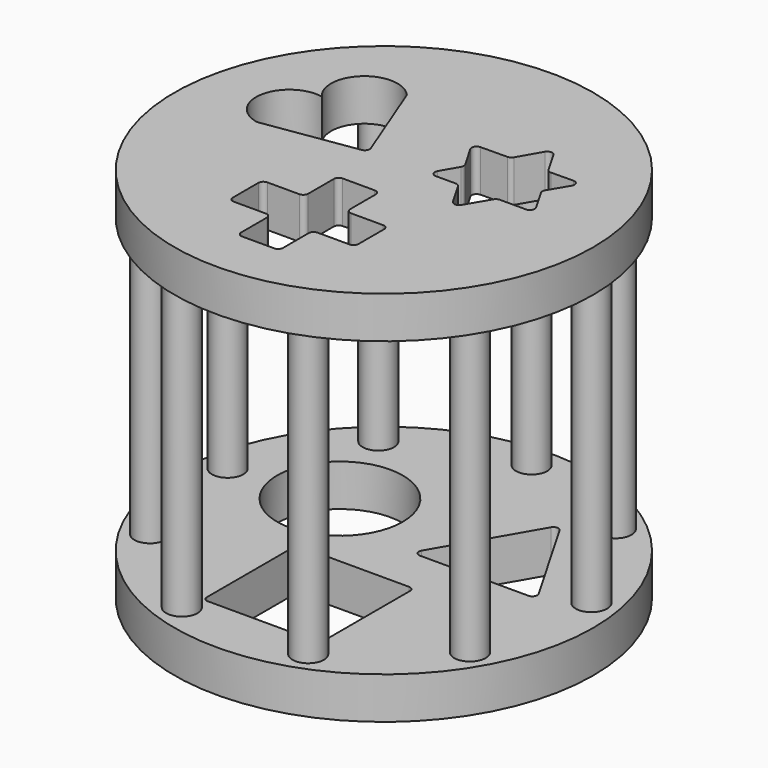
from build123d import *

# Parameters (mm, degrees)
F0_R      = 63.5
F0_R_2    = 19.05
F1_DEPTH  = 12.7
F2_R      = 4.7625
F3_DEPTH  = 6.35
F4_R      = 4.7625
F5_DEPTH  = 101.6
F7_COUNT  = 9
F7_ANGLE  = 320
F9_R      = 63.5
F10_DEPTH = 12.7
F11_R     = 4.7625
F12_DEPTH = 6.35


# Not quite as in the source:
# - a length typed as a fraction of an inch, garbled in the dataset ("3 / 203.2 mm" for 3/8 in), is restored


with BuildPart() as f1:
    # F0 (on Top) → F1 (new body)
    with BuildSketch(Plane.XY):
        Circle(F0_R)
        with BuildLine():
            Line((-17.78, -44.855), (-17.78, -12.295))
            ThreePointArc((-17.78, -12.295), (-17.3406601718, -11.2343398282), (-16.28, -10.795))
            Line((-16.28, -10.795), (16.28, -10.795))
            ThreePointArc((16.28, -10.795), (17.3406601718, -11.2343398282), (17.78, -12.295))
            Line((17.78, -12.295), (17.78, -44.855))
            ThreePointArc((17.78, -44.855), (17.3406601718, -45.9156601718), (16.28, -46.355))
            Line((16.28, -46.355), (-16.28, -46.355))
            ThreePointArc((-16.28, -46.355), (-17.3406601718, -45.9156601718), (-17.78, -44.855))
        make_face(mode=Mode.SUBTRACT)
        with Locations((-24.7466759131, 14.2875)):
            Circle(F0_R_2, mode=Mode.SUBTRACT)
        with BuildLine():
            ThreePointArc((8.2947521245, 3.2889773719), (6.9957140188, 4.0389773719), (6.9957140188, 5.5389773719))
            Line((6.9957140188, 5.5389773719), (23.4476378075, 34.0345452561))
            ThreePointArc((23.4476378075, 34.0345452561), (24.7466759131, 34.7845452561), (26.0457140188, 34.0345452561))
            Line((26.0457140188, 34.0345452561), (42.4976378075, 5.5389773719))
            ThreePointArc((42.4976378075, 5.5389773719), (42.4976378075, 4.0389773719), (41.1985997018, 3.2889773719))
            Line((41.1985997018, 3.2889773719), (8.2947521245, 3.2889773719))
        make_face(mode=Mode.SUBTRACT)
    extrude(amount=F1_DEPTH)

    # F2 (on face) → F3 (cut)
    with BuildSketch(Plane.XY.offset(12.7)):
        with Locations((0, 56)):
            Circle(F2_R)
        with Locations((-35.9961061424, 42.8984888147)):
            Circle(F2_R)
        with Locations((-55.1492341687, 9.7242979493)):
            Circle(F2_R)
        with Locations((-48.4974226119, -28)):
            Circle(F2_R)
        with Locations((-19.1531280262, -52.622786764)):
            Circle(F2_R)
        with Locations((19.1531280262, -52.622786764)):
            Circle(F2_R)
        with Locations((48.4974226119, -28)):
            Circle(F2_R)
        with Locations((55.1492341687, 9.7242979493)):
            Circle(F2_R)
        with Locations((35.9961061424, 42.8984888147)):
            Circle(F2_R)
    extrude(amount=-F3_DEPTH, mode=Mode.SUBTRACT)


with BuildPart() as f5:
    # F4 (on face) → F5 (new body)
    with BuildSketch(Plane.XY.offset(6.35)):
        with Locations((0, 56)):
            Circle(F4_R)
    extrude(amount=F5_DEPTH)


with BuildPart() as f7_1:
    # F7: instance of F5
    add(f5.part.rotate(Axis((0, 0, 35.4298762977), (0, 0, 1)), 1 * F7_ANGLE / (F7_COUNT - 1)))


with BuildPart() as f7_2:
    # F7: instance of F5
    add(f5.part.rotate(Axis((0, 0, 35.4298762977), (0, 0, 1)), 2 * F7_ANGLE / (F7_COUNT - 1)))


with BuildPart() as f7_3:
    # F7: instance of F5
    add(f5.part.rotate(Axis((0, 0, 35.4298762977), (0, 0, 1)), 3 * F7_ANGLE / (F7_COUNT - 1)))


with BuildPart() as f7_4:
    # F7: instance of F5
    add(f5.part.rotate(Axis((0, 0, 35.4298762977), (0, 0, 1)), 4 * F7_ANGLE / (F7_COUNT - 1)))


with BuildPart() as f7_5:
    # F7: instance of F5
    add(f5.part.rotate(Axis((0, 0, 35.4298762977), (0, 0, 1)), 5 * F7_ANGLE / (F7_COUNT - 1)))


with BuildPart() as f7_6:
    # F7: instance of F5
    add(f5.part.rotate(Axis((0, 0, 35.4298762977), (0, 0, 1)), 6 * F7_ANGLE / (F7_COUNT - 1)))


with BuildPart() as f7_7:
    # F7: instance of F5
    add(f5.part.rotate(Axis((0, 0, 35.4298762977), (0, 0, 1)), 7 * F7_ANGLE / (F7_COUNT - 1)))


with BuildPart() as f7_8:
    # F7: instance of F5
    add(f5.part.rotate(Axis((0, 0, 35.4298762977), (0, 0, 1)), 8 * F7_ANGLE / (F7_COUNT - 1)))


with BuildPart() as f10:
    # F9 (on offset) → F10 (new body)
    with BuildSketch(Plane.XY.offset(101.6)):
        Circle(F9_R)
        with BuildLine():
            ThreePointArc((-6.35, -11.025), (-5.9106601718, -9.9643398282), (-4.85, -9.525))
            Line((-4.85, -9.525), (4.85, -9.525))
            ThreePointArc((4.85, -9.525), (5.9106601718, -9.9643398282), (6.35, -11.025))
            Line((6.35, -11.025), (6.35, -20.725))
            ThreePointArc((6.35, -20.725), (6.7893398282, -21.7856601718), (7.85, -22.225))
            Line((7.85, -22.225), (17.55, -22.225))
            ThreePointArc((17.55, -22.225), (18.6106601718, -22.6643398282), (19.05, -23.725))
            Line((19.05, -23.725), (19.05, -33.425))
            ThreePointArc((19.05, -33.425), (18.6106601718, -34.4856601718), (17.55, -34.925))
            Line((17.55, -34.925), (7.85, -34.925))
            ThreePointArc((7.85, -34.925), (6.7893398282, -35.3643398282), (6.35, -36.425))
            Line((6.35, -36.425), (6.35, -46.125))
            ThreePointArc((6.35, -46.125), (5.9106601718, -47.1856601718), (4.85, -47.625))
            Line((4.85, -47.625), (-4.85, -47.625))
            ThreePointArc((-4.85, -47.625), (-5.9106601718, -47.1856601718), (-6.35, -46.125))
            Line((-6.35, -46.125), (-6.35, -36.425))
            ThreePointArc((-6.35, -36.425), (-6.7893398282, -35.3643398282), (-7.85, -34.925))
            Line((-7.85, -34.925), (-17.55, -34.925))
            ThreePointArc((-17.55, -34.925), (-18.6106601718, -34.4856601718), (-19.05, -33.425))
            Line((-19.05, -33.425), (-19.05, -23.725))
            ThreePointArc((-19.05, -23.725), (-18.6106601718, -22.6643398282), (-17.55, -22.225))
            Line((-17.55, -22.225), (-7.85, -22.225))
            ThreePointArc((-7.85, -22.225), (-6.7893398282, -21.7856601718), (-6.35, -20.725))
            Line((-6.35, -20.725), (-6.35, -11.025))
        make_face(mode=Mode.SUBTRACT)
        with BuildLine():
            ThreePointArc((-9.3414467161, 6.7454026488), (-9.439758788, 5.4500472773), (-10.5124134107, 4.7172288398))
            Line((-10.5124134107, 4.7172288398), (-38.7923117777, 0.3997063912))
            ThreePointArc((-38.7923117777, 0.3997063912), (-46.7750013369, 12.2063190546), (-34.9683886735, 20.1890086138))
            ThreePointArc((-34.9683886735, 20.1890086138), (-33.9584830564, 34.4051798925), (-19.7423117777, 33.3952742754))
            Line((-19.7423117777, 33.3952742754), (-9.3414467161, 6.7454026488))
        make_face(mode=Mode.SUBTRACT)
        with BuildLine():
            Line((20.0025253225, 24.2536795687), (23.9442948534, 31.0810246679))
            ThreePointArc((23.9442948534, 31.0810246679), (25.243332959, 31.8310246679), (26.5423710647, 31.0810246679))
            Line((26.5423710647, 31.0810246679), (30.396885254, 24.4048102536))
            ThreePointArc((30.396885254, 24.4048102536), (30.9534909993, 23.8514322615), (31.7133704873, 23.6549117245))
            Line((31.7133704873, 23.6549117245), (38.4927493842, 23.7337708518))
            ThreePointArc((38.4927493842, 23.7337708518), (39.8092346175, 22.9838723227), (39.8004231773, 21.4688134023))
            Line((39.8004231773, 21.4688134023), (36.3424397213, 15.6371286194))
            ThreePointArc((36.3424397213, 15.6371286194), (36.1326917548, 14.8807934104), (36.3336282812, 14.122069699))
            Line((36.3336282812, 14.122069699), (40.1881424704, 7.4458552847))
            ThreePointArc((40.1881424704, 7.4458552847), (40.1881424704, 5.9458552847), (38.8891043648, 5.1958552847))
            Line((38.8891043648, 5.1958552847), (31.005565303, 5.1958552847))
            ThreePointArc((31.005565303, 5.1958552847), (30.2631329426, 4.9992332768), (29.7153386375, 4.4609142051))
            Line((29.7153386375, 4.4609142051), (25.5575192448, -2.5510025352))
            ThreePointArc((25.5575192448, -2.5510025352), (24.2585688679, -3.2859182469), (22.9682544736, -2.5359436148))
            Line((22.9682544736, -2.5359436148), (18.9373109995, 4.4458552847))
            ThreePointArc((18.9373109995, 4.4458552847), (18.3882728938, 4.9948933904), (17.6382728938, 5.1958552847))
            Line((17.6382728938, 5.1958552847), (11.5975615533, 5.1958552847))
            ThreePointArc((11.5975615533, 5.1958552847), (10.2985234476, 5.9458552847), (10.2985234476, 7.4458552847))
            Line((10.2985234476, 7.4458552847), (13.3188791179, 12.6772647626))
            ThreePointArc((13.3188791179, 12.6772647626), (13.5198410122, 13.4272647626), (13.3188791179, 14.1772647626))
            Line((13.3188791179, 14.1772647626), (9.2879356438, 21.1590636621))
            ThreePointArc((9.2879356438, 21.1590636621), (9.2835957574, 22.6514960225), (10.5695266218, 23.4089621913))
            Line((10.5695266218, 23.4089621913), (18.7209343445, 23.5037810396))
            ThreePointArc((18.7209343445, 23.5037810396), (19.4610294885, 23.709025288), (20.0025253225, 24.2536795687))
        make_face(mode=Mode.SUBTRACT)
    extrude(amount=F10_DEPTH)

    # F11 (on face) → F12 (cut)
    with BuildSketch(Plane(origin=(0, 0, 101.6), x_dir=(1, 0, 0), z_dir=(0, 0, -1))):
        with Locations((-19.1531280262, 52.622786764)):
            Circle(F11_R)
        with Locations((-48.4974226119, 28)):
            Circle(F11_R)
        with Locations((-55.1492341687, -9.7242979493)):
            Circle(F11_R)
        with Locations((-35.9961061424, -42.8984888147)):
            Circle(F11_R)
        with Locations((0, -56)):
            Circle(F11_R)
        with Locations((35.9961061424, -42.8984888147)):
            Circle(F11_R)
        with Locations((55.1492341687, -9.7242979493)):
            Circle(F11_R)
        with Locations((48.4974226119, 28)):
            Circle(F11_R)
        with Locations((19.1531280262, 52.622786764)):
            Circle(F11_R)
    extrude(amount=-F12_DEPTH, mode=Mode.SUBTRACT)


solid = Compound([f1.part, f5.part, f7_1.part, f7_2.part, f7_3.part, f7_4.part, f7_5.part, f7_6.part, f7_7.part, f7_8.part, f10.part])
